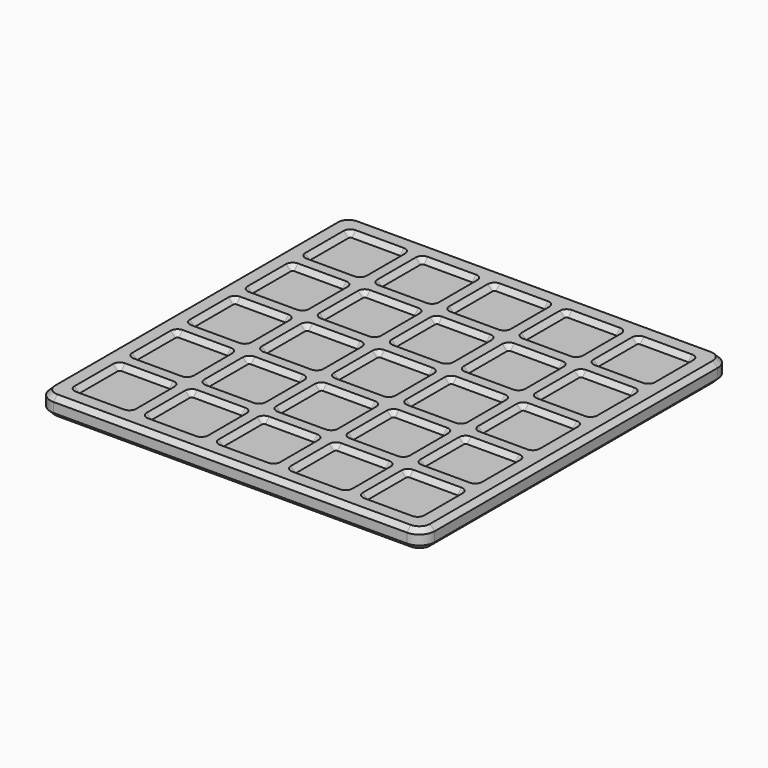
from build123d import *

# Parameters (mm, degrees)
F0_W     = 127
F0_H     = 127
F0_W_2   = 17.145
F0_H_2   = 17.145
F1_DEPTH = 6.35
F2_DEPTH = 4.7625
F3_R     = 0.635
F4_R     = 5.08
F5_SIZE  = 1.58749


# Not quite as in the source:
# - a fillet or chamfer is up to 0.001 mm smaller than in the source, because OpenCascade refuses the exact size


with BuildPart() as f1:
    # F0 (on Top) → F1 (new body)
    with BuildSketch(Plane.XY):
        Rectangle(F0_W, F0_H)
        with Locations((-47.625, -47.625)):
            Rectangle(F0_W_2, F0_H_2, mode=Mode.SUBTRACT)
        with Locations((-23.8125, -47.625)):
            Rectangle(F0_W_2, F0_H_2, mode=Mode.SUBTRACT)
        with Locations((-47.625, -23.8125)):
            Rectangle(F0_W_2, F0_H_2, mode=Mode.SUBTRACT)
        with Locations((-23.8125, -23.8125)):
            Rectangle(F0_W_2, F0_H_2, mode=Mode.SUBTRACT)
        with Locations((0, -47.625)):
            Rectangle(F0_W_2, F0_H_2, mode=Mode.SUBTRACT)
        with Locations((23.8125, -47.625)):
            Rectangle(F0_W_2, F0_H_2, mode=Mode.SUBTRACT)
        with Locations((47.625, -47.625)):
            Rectangle(F0_W_2, F0_H_2, mode=Mode.SUBTRACT)
        with Locations((0, -23.8125)):
            Rectangle(F0_W_2, F0_H_2, mode=Mode.SUBTRACT)
        with Locations((23.8125, -23.8125)):
            Rectangle(F0_W_2, F0_H_2, mode=Mode.SUBTRACT)
        with Locations((47.625, -23.8125)):
            Rectangle(F0_W_2, F0_H_2, mode=Mode.SUBTRACT)
        with Locations((-47.625, 0)):
            Rectangle(F0_W_2, F0_H_2, mode=Mode.SUBTRACT)
        with Locations((-47.625, 23.8125)):
            Rectangle(F0_W_2, F0_H_2, mode=Mode.SUBTRACT)
        with Locations((-23.8125, 0)):
            Rectangle(F0_W_2, F0_H_2, mode=Mode.SUBTRACT)
        with Locations((-23.8125, 23.8125)):
            Rectangle(F0_W_2, F0_H_2, mode=Mode.SUBTRACT)
        with Locations((-47.625, 47.625)):
            Rectangle(F0_W_2, F0_H_2, mode=Mode.SUBTRACT)
        with Locations((-23.8125, 47.625)):
            Rectangle(F0_W_2, F0_H_2, mode=Mode.SUBTRACT)
        Rectangle(F0_W_2, F0_H_2, mode=Mode.SUBTRACT)
        with Locations((23.8125, 0)):
            Rectangle(F0_W_2, F0_H_2, mode=Mode.SUBTRACT)
        with Locations((0, 23.8125)):
            Rectangle(F0_W_2, F0_H_2, mode=Mode.SUBTRACT)
        with Locations((23.8125, 23.8125)):
            Rectangle(F0_W_2, F0_H_2, mode=Mode.SUBTRACT)
        with Locations((47.625, 0)):
            Rectangle(F0_W_2, F0_H_2, mode=Mode.SUBTRACT)
        with Locations((47.625, 23.8125)):
            Rectangle(F0_W_2, F0_H_2, mode=Mode.SUBTRACT)
        with Locations((0, 47.625)):
            Rectangle(F0_W_2, F0_H_2, mode=Mode.SUBTRACT)
        with Locations((23.8125, 47.625)):
            Rectangle(F0_W_2, F0_H_2, mode=Mode.SUBTRACT)
        with Locations((47.625, 47.625)):
            Rectangle(F0_W_2, F0_H_2, mode=Mode.SUBTRACT)
    extrude(amount=F1_DEPTH)

    # F0 (on Top) → F2 (join)
    with BuildSketch(Plane.XY):
        with Locations((-47.625, -47.625)):
            Rectangle(F0_W_2, F0_H_2)
        with Locations((-47.625, -23.8125)):
            Rectangle(F0_W_2, F0_H_2)
        with Locations((-47.625, 0)):
            Rectangle(F0_W_2, F0_H_2)
        with Locations((-47.625, 23.8125)):
            Rectangle(F0_W_2, F0_H_2)
        with Locations((-47.625, 47.625)):
            Rectangle(F0_W_2, F0_H_2)
        with Locations((-23.8125, 47.625)):
            Rectangle(F0_W_2, F0_H_2)
        with Locations((-23.8125, 23.8125)):
            Rectangle(F0_W_2, F0_H_2)
        with Locations((-23.8125, 0)):
            Rectangle(F0_W_2, F0_H_2)
        with Locations((-23.8125, -23.8125)):
            Rectangle(F0_W_2, F0_H_2)
        with Locations((-23.8125, -47.625)):
            Rectangle(F0_W_2, F0_H_2)
        with Locations((0, -47.625)):
            Rectangle(F0_W_2, F0_H_2)
        with Locations((0, -23.8125)):
            Rectangle(F0_W_2, F0_H_2)
        Rectangle(F0_W_2, F0_H_2)
        with Locations((0, 23.8125)):
            Rectangle(F0_W_2, F0_H_2)
        with Locations((0, 47.625)):
            Rectangle(F0_W_2, F0_H_2)
        with Locations((23.8125, 47.625)):
            Rectangle(F0_W_2, F0_H_2)
        with Locations((23.8125, 23.8125)):
            Rectangle(F0_W_2, F0_H_2)
        with Locations((23.8125, 0)):
            Rectangle(F0_W_2, F0_H_2)
        with Locations((23.8125, -23.8125)):
            Rectangle(F0_W_2, F0_H_2)
        with Locations((23.8125, -47.625)):
            Rectangle(F0_W_2, F0_H_2)
        with Locations((47.625, -47.625)):
            Rectangle(F0_W_2, F0_H_2)
        with Locations((47.625, -23.8125)):
            Rectangle(F0_W_2, F0_H_2)
        with Locations((47.625, 0)):
            Rectangle(F0_W_2, F0_H_2)
        with Locations((47.625, 47.625)):
            Rectangle(F0_W_2, F0_H_2)
        with Locations((47.625, 23.8125)):
            Rectangle(F0_W_2, F0_H_2)
    extrude(amount=F2_DEPTH)

    # F3
    f3_edges = [f1.edges().sort_by_distance(p)[0] for p in [
        (-56.1975, -39.0525, 5.55625),
        (-32.385, -15.24, 5.55625),
        (-32.385, 8.5725, 5.55625),
        (-32.385, 32.385, 5.55625),
        (-56.1975, 8.5725, 5.55625),
        (-8.5725, 8.5725, 5.55625),
        (-8.5725, -15.24, 5.55625),
        (-8.5725, -39.0525, 5.55625),
        (-32.385, -39.0525, 5.55625),
        (-8.5725, 32.385, 5.55625),
        (-8.5725, 56.1975, 5.55625),
        (-32.385, 56.1975, 5.55625),
        (-56.1975, -15.24, 5.55625),
        (-56.1975, 32.385, 5.55625),
        (-56.1975, 56.1975, 5.55625),
        (15.24, 56.1975, 5.55625),
        (39.0525, 56.1975, 5.55625),
        (39.0525, 32.385, 5.55625),
        (15.24, 32.385, 5.55625),
        (15.24, 8.5725, 5.55625),
        (39.0525, 8.5725, 5.55625),
        (39.0525, -15.24, 5.55625),
        (15.24, -15.24, 5.55625),
        (15.24, -39.0525, 5.55625),
        (39.0525, -39.0525, 5.55625),
        (56.1975, -56.1975, 5.55625),
        (56.1975, -32.385, 5.55625),
        (32.385, -32.385, 5.55625),
        (32.385, -56.1975, 5.55625),
        (-15.24, -32.385, 5.55625),
        (8.5725, -32.385, 5.55625),
        (8.5725, -56.1975, 5.55625),
        (-15.24, -56.1975, 5.55625),
        (-39.0525, -56.1975, 5.55625),
        (8.5725, 39.0525, 5.55625),
        (8.5725, 15.24, 5.55625),
        (8.5725, -8.5725, 5.55625),
        (32.385, -8.5725, 5.55625),
        (56.1975, -8.5725, 5.55625),
        (56.1975, 15.24, 5.55625),
        (56.1975, 39.0525, 5.55625),
        (32.385, 39.0525, 5.55625),
        (32.385, 15.24, 5.55625),
        (-15.24, 39.0525, 5.55625),
        (-15.24, 15.24, 5.55625),
        (-15.24, -8.5725, 5.55625),
        (-39.0525, -32.385, 5.55625),
        (-39.0525, -8.5725, 5.55625),
        (-39.0525, 15.24, 5.55625),
        (-39.0525, 39.0525, 5.55625),
        (-56.1975, 15.24, 5.55625),
        (-56.1975, 39.0525, 5.55625),
        (-56.1975, -8.5725, 5.55625),
        (-56.1975, -32.385, 5.55625),
        (-56.1975, -56.1975, 5.55625),
        (-32.385, -56.1975, 5.55625),
        (-32.385, -32.385, 5.55625),
        (-32.385, -8.5725, 5.55625),
        (-32.385, 15.24, 5.55625),
        (-32.385, 39.0525, 5.55625),
        (-8.5725, -56.1975, 5.55625),
        (-8.5725, -32.385, 5.55625),
        (-8.5725, -8.5725, 5.55625),
        (-8.5725, 15.24, 5.55625),
        (-8.5725, 39.0525, 5.55625),
        (15.24, 39.0525, 5.55625),
        (15.24, 15.24, 5.55625),
        (15.24, -8.5725, 5.55625),
        (15.24, -32.385, 5.55625),
        (15.24, -56.1975, 5.55625),
        (39.0525, -56.1975, 5.55625),
        (39.0525, -32.385, 5.55625),
        (39.0525, -8.5725, 5.55625),
        (39.0525, 15.24, 5.55625),
        (39.0525, 39.0525, 5.55625),
        (-39.0525, 56.1975, 5.55625),
        (-39.0525, 8.5725, 5.55625),
        (-39.0525, -15.24, 5.55625),
        (-39.0525, -39.0525, 5.55625),
        (-15.24, -39.0525, 5.55625),
        (-15.24, -15.24, 5.55625),
        (-15.24, 8.5725, 5.55625),
        (-15.24, 32.385, 5.55625),
        (-15.24, 56.1975, 5.55625),
        (8.5725, 56.1975, 5.55625),
        (8.5725, 32.385, 5.55625),
        (8.5725, 8.5725, 5.55625),
        (-39.0525, 32.385, 5.55625),
        (8.5725, -15.24, 5.55625),
        (8.5725, -39.0525, 5.55625),
        (32.385, -39.0525, 5.55625),
        (32.385, -15.24, 5.55625),
        (32.385, 8.5725, 5.55625),
        (32.385, 32.385, 5.55625),
        (56.1975, 56.1975, 5.55625),
        (56.1975, -15.24, 5.55625),
        (56.1975, -39.0525, 5.55625),
        (56.1975, 8.5725, 5.55625),
        (56.1975, 32.385, 5.55625),
        (32.385, 56.1975, 5.55625),
    ]]
    fillet(f3_edges, radius=F3_R)

    # F4
    f4_edges = [f1.edges().sort_by_distance(p)[0] for p in [
        (-63.5, 63.5, 3.175),
        (63.5, 63.5, 3.175),
        (63.5, -63.5, 3.175),
        (-63.5, -63.5, 3.175),
    ]]
    fillet(f4_edges, radius=F4_R)

    # F5 (size 1.5875 in the source; OpenCascade refuses exactly that, so slightly less here)
    f5_edges = [f1.edges().sort_by_distance(p)[0] for p in [
        (63.5, 0, 6.35),
        (62.012102, -62.012102, 6.35),
        (62.012102, 62.012102, 6.35),
        (0, -63.5, 6.35),
        (0, 63.5, 6.35),
        (-62.012102, -62.012102, 6.35),
        (-62.012102, 62.012102, 6.35),
        (-63.5, 0, 6.35),
        (-47.625, -39.0525, 6.35),
        (-56.011513, -39.238487, 6.35),
        (-39.238487, -39.238487, 6.35),
        (-56.1975, -47.625, 6.35),
        (-39.0525, -47.625, 6.35),
        (-56.011513, -56.011513, 6.35),
        (-39.238487, -56.011513, 6.35),
        (-47.625, -56.1975, 6.35),
        (-23.8125, -39.0525, 6.35),
        (-32.199013, -39.238487, 6.35),
        (-15.425987, -39.238487, 6.35),
        (-32.385, -47.625, 6.35),
        (-15.24, -47.625, 6.35),
        (-32.199013, -56.011513, 6.35),
        (-15.425987, -56.011513, 6.35),
        (-23.8125, -56.1975, 6.35),
        (-47.625, -15.24, 6.35),
        (-56.011513, -15.425987, 6.35),
        (-39.238487, -15.425987, 6.35),
        (-56.1975, -23.8125, 6.35),
        (-39.0525, -23.8125, 6.35),
        (-56.011513, -32.199013, 6.35),
        (-39.238487, -32.199013, 6.35),
        (-47.625, -32.385, 6.35),
        (-23.8125, -15.24, 6.35),
        (-32.199013, -15.425987, 6.35),
        (-15.425987, -15.425987, 6.35),
        (-32.385, -23.8125, 6.35),
        (-15.24, -23.8125, 6.35),
        (-32.199013, -32.199013, 6.35),
        (-15.425987, -32.199013, 6.35),
        (-23.8125, -32.385, 6.35),
        (-8.5725, -47.625, 6.35),
        (-8.386513, -56.011513, 6.35),
        (-8.386513, -39.238487, 6.35),
        (0, -56.1975, 6.35),
        (0, -39.0525, 6.35),
        (8.386513, -56.011513, 6.35),
        (8.386513, -39.238487, 6.35),
        (8.5725, -47.625, 6.35),
        (23.8125, -39.0525, 6.35),
        (15.425987, -39.238487, 6.35),
        (32.199013, -39.238487, 6.35),
        (15.24, -47.625, 6.35),
        (32.385, -47.625, 6.35),
        (15.425987, -56.011513, 6.35),
        (32.199013, -56.011513, 6.35),
        (23.8125, -56.1975, 6.35),
        (56.1975, -47.625, 6.35),
        (56.011513, -39.238487, 6.35),
        (56.011513, -56.011513, 6.35),
        (47.625, -39.0525, 6.35),
        (47.625, -56.1975, 6.35),
        (39.238487, -39.238487, 6.35),
        (39.238487, -56.011513, 6.35),
        (39.0525, -47.625, 6.35),
        (-8.5725, -23.8125, 6.35),
        (-8.386513, -32.199013, 6.35),
        (-8.386513, -15.425987, 6.35),
        (0, -32.385, 6.35),
        (0, -15.24, 6.35),
        (8.386513, -32.199013, 6.35),
        (8.386513, -15.425987, 6.35),
        (8.5725, -23.8125, 6.35),
        (23.8125, -15.24, 6.35),
        (15.425987, -15.425987, 6.35),
        (32.199013, -15.425987, 6.35),
        (15.24, -23.8125, 6.35),
        (32.385, -23.8125, 6.35),
        (15.425987, -32.199013, 6.35),
        (32.199013, -32.199013, 6.35),
        (23.8125, -32.385, 6.35),
        (56.1975, -23.8125, 6.35),
        (56.011513, -15.425987, 6.35),
        (56.011513, -32.199013, 6.35),
        (47.625, -15.24, 6.35),
        (47.625, -32.385, 6.35),
        (39.238487, -15.425987, 6.35),
        (39.238487, -32.199013, 6.35),
        (39.0525, -23.8125, 6.35),
        (-56.1975, 0, 6.35),
        (-56.011513, -8.386513, 6.35),
        (-56.011513, 8.386513, 6.35),
        (-47.625, -8.5725, 6.35),
        (-47.625, 8.5725, 6.35),
        (-39.238487, -8.386513, 6.35),
        (-39.238487, 8.386513, 6.35),
        (-39.0525, 0, 6.35),
        (-56.1975, 23.8125, 6.35),
        (-56.011513, 15.425987, 6.35),
        (-56.011513, 32.199013, 6.35),
        (-47.625, 15.24, 6.35),
        (-47.625, 32.385, 6.35),
        (-39.238487, 15.425987, 6.35),
        (-39.238487, 32.199013, 6.35),
        (-39.0525, 23.8125, 6.35),
        (-32.385, 0, 6.35),
        (-32.199013, -8.386513, 6.35),
        (-32.199013, 8.386513, 6.35),
        (-23.8125, -8.5725, 6.35),
        (-23.8125, 8.5725, 6.35),
        (-15.425987, -8.386513, 6.35),
        (-15.425987, 8.386513, 6.35),
        (-15.24, 0, 6.35),
        (-32.385, 23.8125, 6.35),
        (-32.199013, 15.425987, 6.35),
        (-32.199013, 32.199013, 6.35),
        (-23.8125, 15.24, 6.35),
        (-23.8125, 32.385, 6.35),
        (-15.425987, 15.425987, 6.35),
        (-15.425987, 32.199013, 6.35),
        (-15.24, 23.8125, 6.35),
        (-47.625, 56.1975, 6.35),
        (-56.011513, 56.011513, 6.35),
        (-39.238487, 56.011513, 6.35),
        (-56.1975, 47.625, 6.35),
        (-39.0525, 47.625, 6.35),
        (-56.011513, 39.238487, 6.35),
        (-39.238487, 39.238487, 6.35),
        (-47.625, 39.0525, 6.35),
        (-23.8125, 56.1975, 6.35),
        (-32.199013, 56.011513, 6.35),
        (-15.425987, 56.011513, 6.35),
        (-32.385, 47.625, 6.35),
        (-15.24, 47.625, 6.35),
        (-32.199013, 39.238487, 6.35),
        (-15.425987, 39.238487, 6.35),
        (-23.8125, 39.0525, 6.35),
        (0, 8.5725, 6.35),
        (-8.386513, 8.386513, 6.35),
        (8.386513, 8.386513, 6.35),
        (-8.5725, 0, 6.35),
        (8.5725, 0, 6.35),
        (-8.386513, -8.386513, 6.35),
        (8.386513, -8.386513, 6.35),
        (0, -8.5725, 6.35),
        (23.8125, 8.5725, 6.35),
        (15.425987, 8.386513, 6.35),
        (32.199013, 8.386513, 6.35),
        (15.24, 0, 6.35),
        (32.385, 0, 6.35),
        (15.425987, -8.386513, 6.35),
        (32.199013, -8.386513, 6.35),
        (23.8125, -8.5725, 6.35),
        (-8.5725, 23.8125, 6.35),
        (-8.386513, 15.425987, 6.35),
        (-8.386513, 32.199013, 6.35),
        (0, 15.24, 6.35),
        (0, 32.385, 6.35),
        (8.386513, 15.425987, 6.35),
        (8.386513, 32.199013, 6.35),
        (8.5725, 23.8125, 6.35),
        (15.24, 23.8125, 6.35),
        (15.425987, 15.425987, 6.35),
        (15.425987, 32.199013, 6.35),
        (23.8125, 15.24, 6.35),
        (23.8125, 32.385, 6.35),
        (32.199013, 15.425987, 6.35),
        (32.199013, 32.199013, 6.35),
        (32.385, 23.8125, 6.35),
        (47.625, 8.5725, 6.35),
        (39.238487, 8.386513, 6.35),
        (56.011513, 8.386513, 6.35),
        (39.0525, 0, 6.35),
        (56.1975, 0, 6.35),
        (39.238487, -8.386513, 6.35),
        (56.011513, -8.386513, 6.35),
        (47.625, -8.5725, 6.35),
        (39.0525, 23.8125, 6.35),
        (39.238487, 15.425987, 6.35),
        (39.238487, 32.199013, 6.35),
        (47.625, 15.24, 6.35),
        (47.625, 32.385, 6.35),
        (56.011513, 15.425987, 6.35),
        (56.011513, 32.199013, 6.35),
        (56.1975, 23.8125, 6.35),
        (0, 56.1975, 6.35),
        (-8.386513, 56.011513, 6.35),
        (8.386513, 56.011513, 6.35),
        (-8.5725, 47.625, 6.35),
        (8.5725, 47.625, 6.35),
        (-8.386513, 39.238487, 6.35),
        (8.386513, 39.238487, 6.35),
        (0, 39.0525, 6.35),
        (23.8125, 56.1975, 6.35),
        (15.425987, 56.011513, 6.35),
        (32.199013, 56.011513, 6.35),
        (15.24, 47.625, 6.35),
        (32.385, 47.625, 6.35),
        (15.425987, 39.238487, 6.35),
        (32.199013, 39.238487, 6.35),
        (23.8125, 39.0525, 6.35),
        (47.625, 56.1975, 6.35),
        (39.238487, 56.011513, 6.35),
        (56.011513, 56.011513, 6.35),
        (39.0525, 47.625, 6.35),
        (56.1975, 47.625, 6.35),
        (39.238487, 39.238487, 6.35),
        (56.011513, 39.238487, 6.35),
        (47.625, 39.0525, 6.35),
        (0, -63.5, 0),
    ]]
    chamfer(f5_edges, length=F5_SIZE)


solid = f1.part
